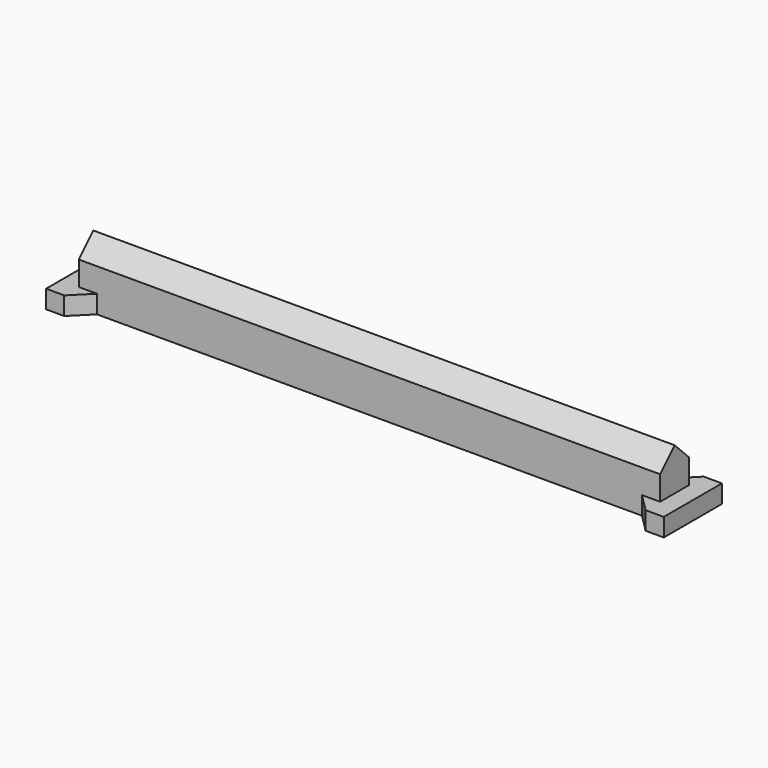
from build123d import *

# Parameters (mm, degrees)
F0_W     = 304.8
F0_H     = 19.05
F1_DEPTH = 31.75
F2_SIZE  = 9.52499
F3_W     = 38.1
F3_H     = 9.525
F4_DEPTH = 9.525
F5_SIZE  = 9.52499


# Not quite as in the source:
# - a fillet or chamfer is up to 0.001 mm smaller than in the source, because OpenCascade refuses the exact size
# - a pattern or mirror of a feature is missing from the dataset's text; its kind, count and spacing are read off the source's solid


with BuildPart() as f1:
    # F0 (on Top) → F1 (new body)
    with BuildSketch(Plane.XY):
        Rectangle(F0_W, F0_H)
    extrude(amount=F1_DEPTH)

    # F2 (size 9.525 in the source; OpenCascade refuses exactly that, so slightly less here)
    f2_edges = [f1.edges().sort_by_distance(p)[0] for p in [
        (0, -9.525, 31.75),
        (0, 9.525, 31.75),
    ]]
    chamfer(f2_edges, length=F2_SIZE)

    # F3 (on face) → F4 (join)
    with BuildSketch(Plane.YZ.offset(152.4)):
        with Locations((0, 4.7625)):
            Rectangle(F3_W, F3_H)
    f4 = extrude(amount=F4_DEPTH)

    # F4_copies: F4 across plane
    add(f4.mirror(Plane(origin=(0, 0, 0), x_dir=(0, 0, -1), z_dir=(-1, 0, 0))))

    # F5 (size 9.525 in the source; OpenCascade refuses exactly that, so slightly less here)
    f5_edges = [f1.edges().sort_by_distance(p)[0] for p in [
        (152.4, -9.525, 4.7625),
        (152.4, 9.525, 4.7625),
        (-152.4, -9.525, 4.7625),
        (-152.4, 9.525, 4.7625),
    ]]
    chamfer(f5_edges, length=F5_SIZE)


solid = f1.part
